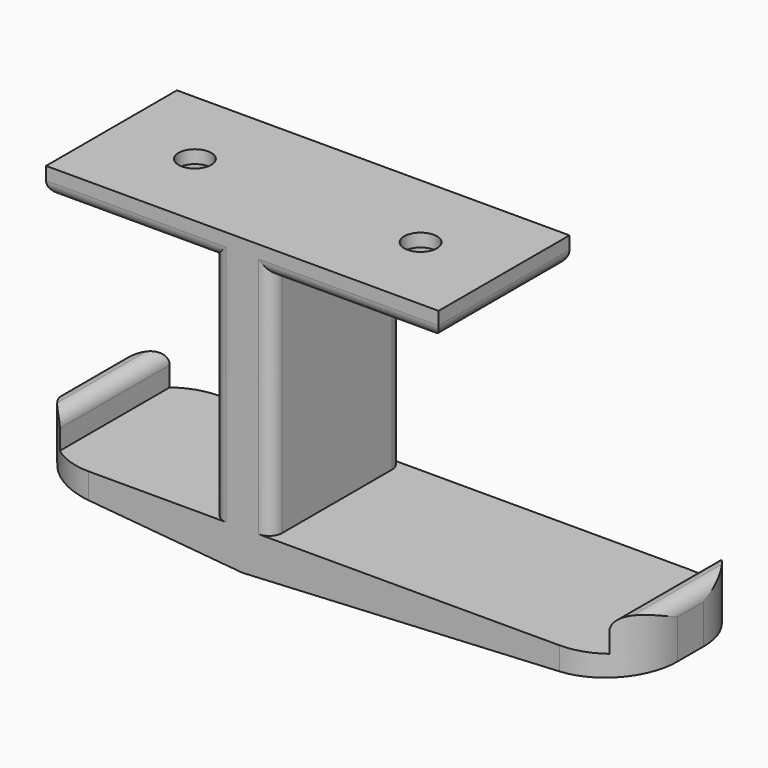
from build123d import *

# Parameters (mm, degrees)
F1_DEPTH       = 12.5
F3_D           = 5
F3_DEPTH       = 12
F3_CBORE_D     = 10
F3_CBORE_DEPTH = 2
F3_TIP         = 1.5021515476
F4_R           = 1.99999
F5_T1_DEPTH    = 56.00001


# Not quite as in the source:
# - a fillet or chamfer that OpenCascade refuses, or shapes differently, is made with other operations: its cross-section is extruded or revolved along the edge and cut away or added
# - a fillet or chamfer is up to 0.001 mm smaller than in the source, because OpenCascade refuses the exact size


with BuildPart() as f1:
    # F0 (on Front) → F1 (new body, symmetric)
    with BuildSketch(Plane.XZ):
        Polygon((54.5, -34), (54.5, -39), (4.5, -39), (4.5, -4), (30, -4), (30, 0), (-30, 0), (-30, -4), (-4.5, -4), (-4.5, -39), (-29.5, -39), (-29.5, -34), (-33.5, -34), (-33.5, -42), (0, -45), (58.5, -42), (58.5, -34), align=None)
    extrude(amount=F1_DEPTH, both=True)

    # F3
    with Locations(Plane(origin=(0, 0, -4), x_dir=(1, 0, 0), z_dir=(0, 0, -1))):
        with Locations((17.25, 0), (-17.25, 0)):
            CounterBoreHole(F3_D / 2, F3_CBORE_D / 2, F3_CBORE_DEPTH, depth=F3_DEPTH)
            with Locations((0, 0, -(F3_DEPTH + F3_TIP / 2))):  # 118° drill point
                Cone(0, F3_D / 2, F3_TIP, mode=Mode.SUBTRACT)

    # F4 (radius 2 in the source; OpenCascade refuses exactly that, so slightly less here)
    f4_edges = [f1.edges().sort_by_distance(p)[0] for p in [
        (58.5, 0, -34),
        (54.5, 0, -34),
        (-29.5, 0, -34),
        (-33.5, 0, -34),
        (30, 0, -4),
        (17.25, -12.5, -4),
        (-17.25, -12.5, -4),
        (-30, 0, -4),
        (-17.25, 12.5, -4),
        (-4.5, 12.5, -21.5),
        (4.5, 12.5, -21.5),
        (-4.5, -12.5, -21.5),
        (4.5, -12.5, -21.5),
        (17.25, 12.5, -4),
    ]]
    fillet(f4_edges, radius=F4_R)

    # F5: fillet of radius 10 on 4 edges, made by hand

    # F5_s2 → F5_t1 (cut)
    with BuildSketch(Plane.XY.offset(-67)):
        with BuildLine():
            ThreePointArc((48.5, 12.5), (55.5710678119, 9.5710678119), (58.5, 2.5))
            Line((58.5, 2.5), (58.5, 12.5))
            Line((58.5, 12.5), (48.5, 12.5))
        make_face()
        with BuildLine():
            ThreePointArc((48.5, -12.5), (55.5710678119, -9.5710678119), (58.5, -2.5))
            Line((58.5, -2.5), (58.5, -12.5))
            Line((58.5, -12.5), (48.5, -12.5))
        make_face()
        with BuildLine():
            ThreePointArc((-23.5, 12.5), (-30.5710678119, 9.5710678119), (-33.5, 2.5))
            Line((-33.5, 2.5), (-33.5, 12.5))
            Line((-33.5, 12.5), (-23.5, 12.5))
        make_face()
        with BuildLine():
            ThreePointArc((-23.5, -12.5), (-30.5710678119, -9.5710678119), (-33.5, -2.5))
            Line((-33.5, -2.5), (-33.5, -12.5))
            Line((-33.5, -12.5), (-23.5, -12.5))
        make_face()
    extrude(amount=F5_T1_DEPTH, mode=Mode.SUBTRACT)


solid = f1.part
